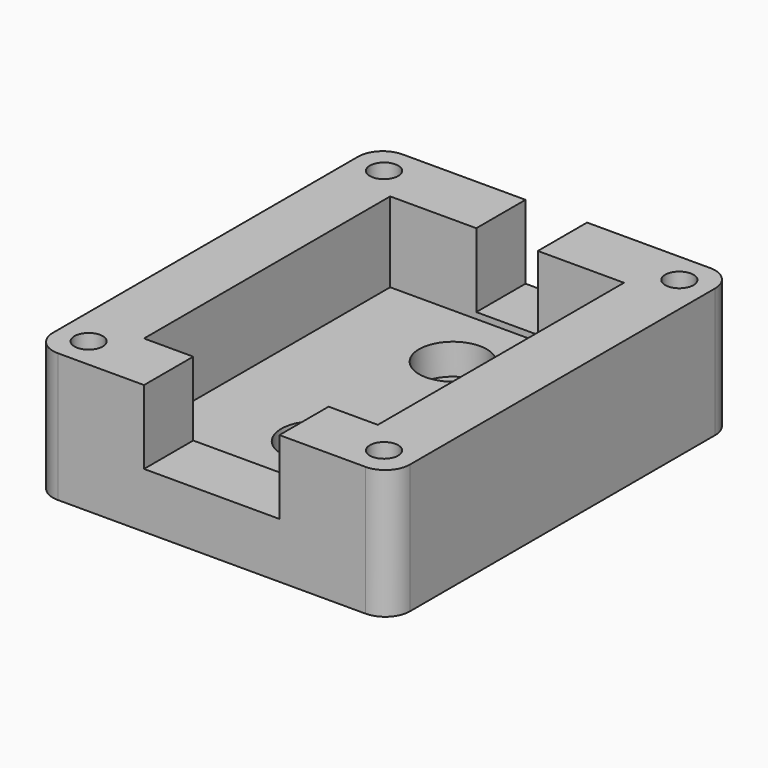
from build123d import *

# Parameters (mm, degrees)
F0_W           = 29
F0_H           = 35
F0_R           = 1.15
F0_W_2         = 19
F0_H_2         = 25
F1_DEPTH       = 6.5
F2_W           = 29
F2_H           = 35
F2_R           = 1.15
F2_W_2         = 19
F2_H_2         = 25
F3_DEPTH       = 4
F4_W           = 11
F4_H           = 5
F4_W_2         = 5
F5_DEPTH       = 6
F6_R           = 2
F8_D           = 2.9
F8_CBORE_D     = 5.5
F8_CBORE_DEPTH = 2.5


with BuildPart() as f1:
    # F0 (on Top) → F1 (new body)
    with BuildSketch(Plane.XY):
        Rectangle(F0_W, F0_H)
        with Locations((-12, -15)):
            Circle(F0_R, mode=Mode.SUBTRACT)
        with Locations((12, -15)):
            Circle(F0_R, mode=Mode.SUBTRACT)
        with Locations((-12, 15)):
            Circle(F0_R, mode=Mode.SUBTRACT)
        Rectangle(F0_W_2, F0_H_2, mode=Mode.SUBTRACT)
        with Locations((12, 15)):
            Circle(F0_R, mode=Mode.SUBTRACT)
    extrude(amount=F1_DEPTH)

    # F2 (on face) → F3 (join)
    with BuildSketch(Plane(origin=(0, 0, 0), x_dir=(1, 0, 0), z_dir=(0, 0, -1))):
        Rectangle(F2_W, F2_H)
        with Locations((-12, -15)):
            Circle(F2_R, mode=Mode.SUBTRACT)
        with Locations((12, -15)):
            Circle(F2_R, mode=Mode.SUBTRACT)
        with Locations((-12, 15)):
            Circle(F2_R, mode=Mode.SUBTRACT)
        Rectangle(F2_W_2, F2_H_2, mode=Mode.SUBTRACT)
        with Locations((12, 15)):
            Circle(F2_R, mode=Mode.SUBTRACT)
        with Locations((-12, 15)):
            Circle(F2_R)
        with Locations((12, 15)):
            Circle(F2_R)
        with Locations((-12, -15)):
            Circle(F2_R)
        Rectangle(F2_W_2, F2_H_2)
        with Locations((12, -15)):
            Circle(F2_R)
    extrude(amount=F3_DEPTH)

    # F4 (on face) → F5 (cut)
    with BuildSketch(Plane.XY.offset(6.5)):
        with Locations((0, -15)):
            Rectangle(F4_W, F4_H)
        with Locations((0, 15)):
            Rectangle(F4_W_2, F4_H)
    extrude(amount=-F5_DEPTH, mode=Mode.SUBTRACT)

    # F6
    f6_edges = [f1.edges().sort_by_distance(p)[0] for p in [
        (-14.5, 17.5, 1.25),
        (14.5, 17.5, 1.25),
        (14.5, -17.5, 1.25),
        (-14.5, -17.5, 1.25),
    ]]
    fillet(f6_edges, radius=F6_R)

    # F8 (through all)
    with Locations(Plane.XY):
        with Locations((0, 7), (0, -7)):
            CounterBoreHole(F8_D / 2, F8_CBORE_D / 2, F8_CBORE_DEPTH)


solid = f1.part
